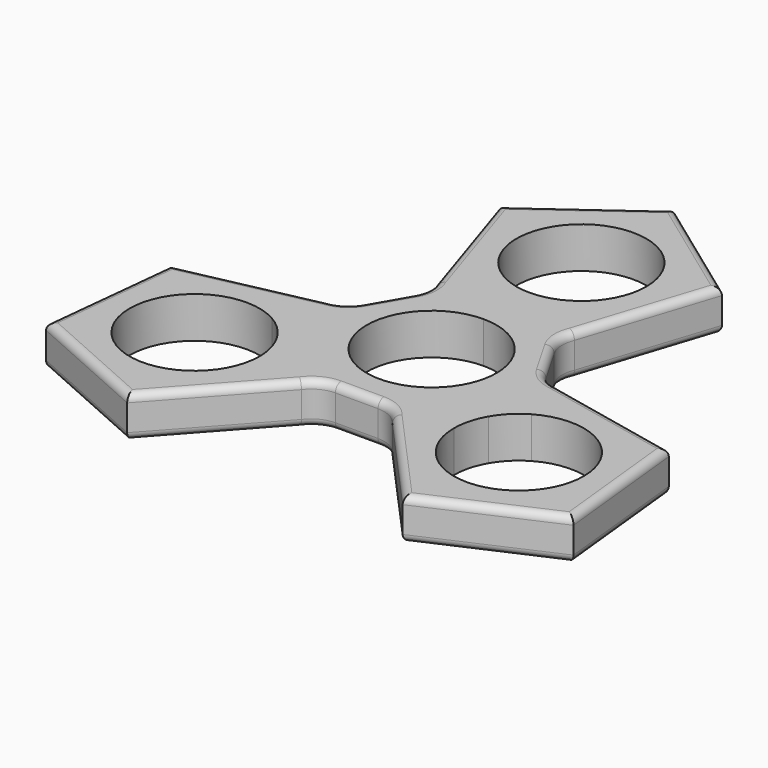
from build123d import *

# Parameters (mm, degrees)
F1_DEPTH    = 6.985
F2_T1_DEPTH = 6.985
F3_R        = 1.27
F4_R        = 1.27


# Not quite as in the source:
# - a fillet or chamfer that OpenCascade refuses, or shapes differently, is made with other operations: its cross-section is extruded or revolved along the edge and cut away or added
# - a feature names something its author has since deleted; it is built from what else it names


with BuildPart() as f1:
    # F0 (on Top) → F1 (new body)
    with BuildSketch(Plane.XY):
        with BuildLine():
            Line((0, 15.6591), (0, 11.0109))
            ThreePointArc((0, 11.0109), (7.785882057, 7.785882057), (11.0109, 0))
            ThreePointArc((11.0109, 0), (10.6357126807, -2.8498306237), (9.5357191185, -5.50545))
            Line((9.5357191185, -5.50545), (13.5611784004, -7.82955))
            Line((13.5611784004, -7.82955), (18.2062211237, 0.2159))
            Line((18.2062211237, 0.2159), (9.2900854465, 15.6591))
            Line((9.2900854465, 15.6591), (0, 15.6591))
        make_face()
        with BuildLine():
            ThreePointArc((-9.5357191185, -5.50545), (-9.5357191185, 5.50545), (0, 11.0109))
            Line((0, 11.0109), (0, 15.6591))
            Line((0, 15.6591), (-9.2900854465, 15.6591))
            Line((-9.2900854465, 15.6591), (-18.2062211237, 0.2159))
            Line((-18.2062211237, 0.2159), (-13.5611784004, -7.82955))
            Line((-13.5611784004, -7.82955), (-9.5357191185, -5.50545))
        make_face()
        with BuildLine():
            Line((13.5611784004, -7.82955), (9.5357191185, -5.50545))
            ThreePointArc((9.5357191185, -5.50545), (0, -11.0109), (-9.5357191185, -5.50545))
            Line((-9.5357191185, -5.50545), (-13.5611784004, -7.82955))
            Line((-13.5611784004, -7.82955), (-8.9161356771, -15.875))
            Line((-8.9161356771, -15.875), (8.9161356771, -15.875))
            Line((8.9161356771, -15.875), (13.5611784004, -7.82955))
        make_face()
        with BuildLine():
            Line((-9.2900854465, 15.6591), (0, 15.6591))
            Line((0, 15.6591), (0, 20.7391))
            ThreePointArc((0, 20.7391), (-2.8498306237, 21.1142873193), (-5.50545, 22.2142808815))
            Line((-5.50545, 22.2142808815), (-9.2900854465, 15.6591))
        make_face()
        with BuildLine():
            Line((0, 20.7391), (0, 15.6591))
            Line((0, 15.6591), (9.2900854465, 15.6591))
            Line((9.2900854465, 15.6591), (5.50545, 22.2142808815))
            ThreePointArc((5.50545, 22.2142808815), (2.8498306237, 21.1142873193), (0, 20.7391))
        make_face()
        with BuildLine():
            Line((18.2062211237, 0.2159), (13.5611784004, -7.82955))
            Line((13.5611784004, -7.82955), (17.9605874516, -10.36955))
            ThreePointArc((17.9605874516, -10.36955), (19.7104245132, -8.089117943), (21.9908565702, -6.3392808815))
            Line((21.9908565702, -6.3392808815), (18.2062211237, 0.2159))
        make_face()
        with BuildLine():
            Line((17.9605874516, -10.36955), (13.5611784004, -7.82955))
            Line((13.5611784004, -7.82955), (8.9161356771, -15.875))
            Line((8.9161356771, -15.875), (16.4854065702, -15.875))
            ThreePointArc((16.4854065702, -15.875), (16.8605938895, -13.0251693763), (17.9605874516, -10.36955))
        make_face()
        with BuildLine():
            Line((-8.9161356771, -15.875), (-13.5611784004, -7.82955))
            Line((-13.5611784004, -7.82955), (-17.9605874516, -10.36955))
            ThreePointArc((-17.9605874516, -10.36955), (-16.8605938895, -13.0251693763), (-16.4854065702, -15.875))
            Line((-16.4854065702, -15.875), (-8.9161356771, -15.875))
        make_face()
        with BuildLine():
            Line((-17.9605874516, -10.36955), (-13.5611784004, -7.82955))
            Line((-13.5611784004, -7.82955), (-18.2062211237, 0.2159))
            Line((-18.2062211237, 0.2159), (-21.9908565702, -6.3392808815))
            ThreePointArc((-21.9908565702, -6.3392808815), (-19.7104245132, -8.089117943), (-17.9605874516, -10.36955))
        make_face()
        with BuildLine():
            Line((5.50545, 22.2142808815), (9.2900854465, 15.6591))
            Line((9.2900854465, 15.6591), (11.6907231639, 15.6591))
            Line((11.6907231639, 15.6591), (18.9159874322, 37.8961768904))
            Line((18.9159874322, 37.8961768904), (0, 51.6394462192))
            Line((0, 51.6394462192), (-18.9159874322, 37.8961768904))
            Line((-18.9159874322, 37.8961768904), (-11.6907231639, 15.6591))
            Line((-11.6907231639, 15.6591), (-9.2900854465, 15.6591))
            Line((-9.2900854465, 15.6591), (-5.50545, 22.2142808815))
            ThreePointArc((-5.50545, 22.2142808815), (-5.50545, 41.2857191185), (11.0109, 31.75))
            ThreePointArc((11.0109, 31.75), (9.5357191185, 26.24455), (5.50545, 22.2142808815))
        make_face()
        with BuildLine():
            Line((16.4854065702, -15.875), (8.9161356771, -15.875))
            Line((8.9161356771, -15.875), (7.7158168185, -17.9540132485))
            Line((7.7158168185, -17.9540132485), (23.3610581773, -35.3298140992))
            Line((23.3610581773, -35.3298140992), (44.7210722631, -25.8197231096))
            Line((44.7210722631, -25.8197231096), (42.2770456095, -2.5663627912))
            Line((42.2770456095, -2.5663627912), (19.4065399823, 2.2949132485))
            Line((19.4065399823, 2.2949132485), (18.2062211237, 0.2159))
            Line((18.2062211237, 0.2159), (21.9908565702, -6.3392808815))
            ThreePointArc((21.9908565702, -6.3392808815), (33.0017565702, -6.3392808815), (38.5072065702, -15.875))
            ThreePointArc((38.5072065702, -15.875), (27.4963065702, -26.8859), (16.4854065702, -15.875))
        make_face()
        with BuildLine():
            Line((-21.9908565702, -6.3392808815), (-18.2062211237, 0.2159))
            Line((-18.2062211237, 0.2159), (-19.4065399823, 2.2949132485))
            Line((-19.4065399823, 2.2949132485), (-42.2770456095, -2.5663627912))
            Line((-42.2770456095, -2.5663627912), (-44.7210722631, -25.8197231096))
            Line((-44.7210722631, -25.8197231096), (-23.3610581773, -35.3298140992))
            Line((-23.3610581773, -35.3298140992), (-7.7158168185, -17.9540132485))
            Line((-7.7158168185, -17.9540132485), (-8.9161356771, -15.875))
            Line((-8.9161356771, -15.875), (-16.4854065702, -15.875))
            ThreePointArc((-16.4854065702, -15.875), (-37.0320256887, -21.38045), (-21.9908565702, -6.3392808815))
        make_face()
    extrude(amount=F1_DEPTH)

    # F2: fillet of radius 5.08 on 6 edges, made by hand

    # F2_s2 → F2_t1 (join)
    with BuildSketch(Plane.XY):
        with BuildLine():
            ThreePointArc((-11.9396642154, 11.0698949536), (-11.2665307911, 13.3347353028), (-11.6907231639, 15.6591))
            Line((-11.6907231639, 15.6591), (-9.2900854465, 15.6591))
            Line((-9.2900854465, 15.6591), (-11.9396642154, 11.0698949536))
        make_face()
        with BuildLine():
            ThreePointArc((-15.5566423547, 4.8051050464), (-17.1814849205, 3.0897342262), (-19.4065399823, 2.2949132485))
            Line((-19.4065399823, 2.2949132485), (-18.2062211237, 0.2159))
            Line((-18.2062211237, 0.2159), (-15.5566423547, 4.8051050464))
        make_face()
        with BuildLine():
            ThreePointArc((-7.7158168185, -17.9540132485), (-5.9149541295, -16.424469529), (-3.6169781393, -15.875))
            Line((-3.6169781393, -15.875), (-8.9161356771, -15.875))
            Line((-8.9161356771, -15.875), (-7.7158168185, -17.9540132485))
        make_face()
        with BuildLine():
            ThreePointArc((3.6169781393, -15.875), (5.9149541295, -16.424469529), (7.7158168185, -17.9540132485))
            Line((7.7158168185, -17.9540132485), (8.9161356771, -15.875))
            Line((8.9161356771, -15.875), (3.6169781393, -15.875))
        make_face()
        with BuildLine():
            ThreePointArc((19.4065399823, 2.2949132485), (17.1814849205, 3.0897342262), (15.5566423547, 4.8051050464))
            Line((15.5566423547, 4.8051050464), (18.2062211237, 0.2159))
            Line((18.2062211237, 0.2159), (19.4065399823, 2.2949132485))
        make_face()
        with BuildLine():
            ThreePointArc((11.9396642154, 11.0698949536), (11.2665307911, 13.3347353028), (11.6907231639, 15.6591))
            Line((11.6907231639, 15.6591), (9.2900854465, 15.6591))
            Line((9.2900854465, 15.6591), (11.9396642154, 11.0698949536))
        make_face()
    extrude(amount=F2_T1_DEPTH)

    # F3
    f3_edges = [f1.edges().sort_by_distance(p)[0] for p in [
        (9.457994, 44.767812, 6.985),
        (15.303355, 26.777638, 6.985),
        (13.748153, 7.9375, 6.985),
        (11.266531, 13.334735, 6.985),
        (17.181485, 3.089734, 6.985),
        (30.841793, -0.135725, 6.985),
        (43.499059, -14.193043, 6.985),
        (34.041065, -30.574769, 6.985),
        (15.538437, -26.641914, 6.985),
        (0, -15.875, 6.985),
        (-5.914954, -16.42447, 6.985),
        (-15.538437, -26.641914, 6.985),
        (-34.041065, -30.574769, 6.985),
        (-43.499059, -14.193043, 6.985),
        (-30.841793, -0.135725, 6.985),
        (-17.181485, 3.089734, 6.985),
        (-13.748153, 7.9375, 6.985),
        (-11.266531, 13.334735, 6.985),
        (-15.303355, 26.777638, 6.985),
        (-9.457994, 44.767812, 6.985),
        (5.914954, -16.42447, 6.985),
    ]]
    fillet(f3_edges, radius=F3_R)

    # F4
    f4_edges = [f1.edges().sort_by_distance(p)[0] for p in [
        (43.499059, -14.193043, 0),
        (34.041065, -30.574769, 0),
        (15.538437, -26.641914, 0),
        (30.841793, -0.135725, 0),
        (15.303355, 26.777638, 0),
        (9.457994, 44.767812, 0),
        (-9.457994, 44.767812, 0),
        (-15.303355, 26.777638, 0),
        (-13.748153, 7.9375, 0),
        (-30.841793, -0.135725, 0),
        (-34.041065, -30.574769, 0),
        (-15.538437, -26.641914, 0),
        (0, -15.875, 0),
        (13.748153, 7.9375, 0),
        (11.266531, 13.334735, 0),
        (-11.266531, 13.334735, 0),
        (17.181485, 3.089734, 0),
        (-17.181485, 3.089734, 0),
        (5.914954, -16.42447, 0),
        (-5.914954, -16.42447, 0),
    ]]
    fillet(f4_edges, radius=F4_R)


solid = f1.part
